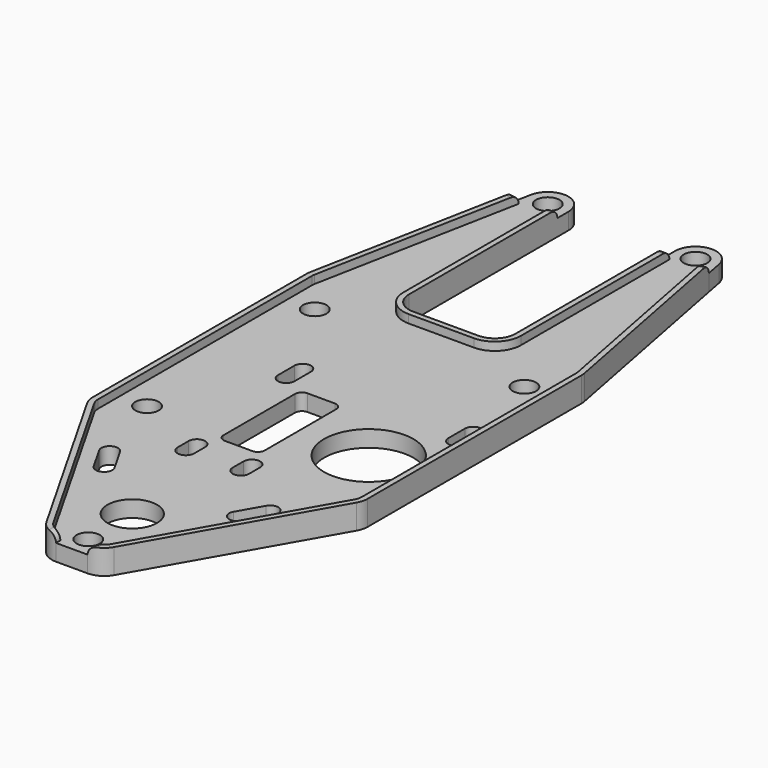
from build123d import *

# Parameters (mm, degrees)
F0_R     = 1.7
F0_R_2   = 3.6
F0_R_3   = 6.5
F1_DEPTH = 2.4
F2_DEPTH = 3.6
F3_R     = 1.19999


# Not quite as in the source:
# - a fillet or chamfer is up to 0.001 mm smaller than in the source, because OpenCascade refuses the exact size


with BuildPart() as f1:
    # F0 (on Top) → F1 (new body)
    with BuildSketch(Plane.XY):
        with BuildLine():
            Line((13.3779826676, 50), (14.1634030533, 50.1520355803))
            Line((14.1634030533, 50.1520355803), (13.6953264465, 52.5701334259))
            ThreePointArc((13.6953264465, 52.5701334259), (12.6591358938, 54.3141305363), (10.75, 55))
            ThreePointArc((10.75, 55), (8.6286796564, 54.1213203436), (7.75, 52))
            Line((7.75, 52), (7.75, 50))
            Line((7.75, 50), (8.55, 50))
            Line((8.55, 50), (8.55, 23))
            ThreePointArc((8.55, 23), (7.4370057685, 20.3129942315), (4.75, 19.2))
            Line((4.75, 19.2), (0, 19.2))
            Line((0, 19.2), (-4.75, 19.2))
            ThreePointArc((-4.75, 19.2), (-7.4370057685, 20.3129942315), (-8.55, 23))
            Line((-8.55, 23), (-8.55, 50))
            Line((-8.55, 50), (-7.75, 50))
            Line((-7.75, 50), (-7.75, 52))
            ThreePointArc((-7.75, 52), (-8.6286796564, 54.1213203436), (-10.75, 55))
            ThreePointArc((-10.75, 55), (-12.6591358938, 54.3141305363), (-13.6953264465, 52.5701334259))
            Line((-13.6953264465, 52.5701334259), (-14.1634030533, 50.1520355803))
            Line((-14.1634030533, 50.1520355803), (-13.3779826676, 50))
            Line((-13.3779826676, 50), (-19.1599060608, 20.1304096433))
            ThreePointArc((-19.1599060608, 20.1304096433), (-19.1899535764, 19.9223197335), (-19.2, 19.7123117976))
            Line((-19.2, 19.7123117976), (-19.2, 0))
            Line((-19.2, 0), (-19.2, -19.2052668078))
            ThreePointArc((-19.2, -19.2052668078), (-19.1266435215, -19.768638206), (-18.9114660616, -20.294439657))
            Line((-18.9114660616, -20.294439657), (-4.2133641117, -46.0891728492))
            ThreePointArc((-4.2133641117, -46.0891728492), (-3.4072983694, -46.9021277912), (-2.3018980501, -47.2))
            Line((-2.3018980501, -47.2), (-2.3018980501, -48))
            Line((-2.3018980501, -48), (0, -48))
            Line((0, -48), (2.3018980501, -48))
            Line((2.3018980501, -48), (2.3018980501, -47.2))
            ThreePointArc((2.3018980501, -47.2), (3.4072983694, -46.9021277912), (4.2133641117, -46.0891728492))
            Line((4.2133641117, -46.0891728492), (18.9114660616, -20.294439657))
            ThreePointArc((18.9114660616, -20.294439657), (19.1266435215, -19.768638206), (19.2, -19.2052668078))
            Line((19.2, -19.2052668078), (19.2, 0))
            Line((19.2, 0), (19.2, 19.7123117976))
            ThreePointArc((19.2, 19.7123117976), (19.1899535764, 19.9223197335), (19.1599060608, 20.1304096433))
            Line((19.1599060608, 20.1304096433), (13.3779826676, 50))
        make_face()
        with BuildLine():
            ThreePointArc((-8.6554840981, -29.4059057186), (-9.1040076685, -31.0426178518), (-10.7407198016, -30.5940942814))
            Line((-10.7407198016, -30.5940942814), (-12.721034073, -27.1187014422))
            ThreePointArc((-12.721034073, -27.1187014422), (-12.2725105026, -25.4819893091), (-10.6357983695, -25.9305128794))
            Line((-10.6357983695, -25.9305128794), (-8.6554840981, -29.4059057186))
        make_face(mode=Mode.SUBTRACT)
        with Locations((-15.25, -15.25)):
            Circle(F0_R, mode=Mode.SUBTRACT)
        with BuildLine():
            Line((-6.2, -21), (-6.2, -19))
            ThreePointArc((-6.2, -19), (-5, -17.8), (-3.8, -19))
            Line((-3.8, -19), (-3.8, -21))
            ThreePointArc((-3.8, -21), (-5, -22.2), (-6.2, -21))
        make_face(mode=Mode.SUBTRACT)
        with BuildLine():
            Line((-8.4, 0), (-8.4, 3))
            ThreePointArc((-8.4, 3), (-7.2, 4.2), (-6, 3))
            Line((-6, 3), (-6, 0))
            ThreePointArc((-6, 0), (-7.2, -1.2), (-8.4, 0))
        make_face(mode=Mode.SUBTRACT)
        with BuildLine():
            ThreePointArc((-4, -2.4), (-3.7071067812, -1.6928932188), (-3, -1.4))
            Line((-3, -1.4), (1, -1.4))
            ThreePointArc((1, -1.4), (1.7071067812, -1.6928932188), (2, -2.4))
            Line((2, -2.4), (2, -15.4))
            ThreePointArc((2, -15.4), (1.7071067812, -16.1071067812), (1, -16.4))
            Line((1, -16.4), (-3, -16.4))
            ThreePointArc((-3, -16.4), (-3.7071067812, -16.1071067812), (-4, -15.4))
            Line((-4, -15.4), (-4, -2.4))
        make_face(mode=Mode.SUBTRACT)
        with Locations((0, -45)):
            Circle(F0_R, mode=Mode.SUBTRACT)
        with Locations((0, -37)):
            Circle(F0_R_2, mode=Mode.SUBTRACT)
        with BuildLine():
            Line((12.721034073, -27.1187014422), (10.7407198016, -30.5940942814))
            ThreePointArc((10.7407198016, -30.5940942814), (9.1040076685, -31.0426178518), (8.6554840981, -29.4059057186))
            Line((8.6554840981, -29.4059057186), (10.6357983695, -25.9305128794))
            ThreePointArc((10.6357983695, -25.9305128794), (12.2725105026, -25.4819893091), (12.721034073, -27.1187014422))
        make_face(mode=Mode.SUBTRACT)
        with BuildLine():
            Line((1.8, -21), (1.8, -19))
            ThreePointArc((1.8, -19), (3, -17.8), (4.2, -19))
            Line((4.2, -19), (4.2, -21))
            ThreePointArc((4.2, -21), (3, -22.2), (1.8, -21))
        make_face(mode=Mode.SUBTRACT)
        with Locations((12, -9)):
            Circle(F0_R_3, mode=Mode.SUBTRACT)
        with BuildLine():
            Line((18.8, 3), (18.8, 0))
            ThreePointArc((18.8, 0), (17.6, -1.2), (16.4, 0))
            Line((16.4, 0), (16.4, 3))
            ThreePointArc((16.4, 3), (17.6, 4.2), (18.8, 3))
        make_face(mode=Mode.SUBTRACT)
        with Locations((-15.25, 15.25)):
            Circle(F0_R, mode=Mode.SUBTRACT)
        with Locations((-10.75, 52)):
            Circle(F0_R, mode=Mode.SUBTRACT)
        with Locations((15.25, 15.25)):
            Circle(F0_R, mode=Mode.SUBTRACT)
        with Locations((10.75, 52)):
            Circle(F0_R, mode=Mode.SUBTRACT)
    extrude(amount=F1_DEPTH)

    # F0 (on Top) → F2 (join)
    with BuildSketch(Plane.XY):
        with BuildLine():
            Line((20, -19.2052668078), (20, 0))
            Line((20, 0), (20, 19.7123117976))
            ThreePointArc((20, 19.7123117976), (19.9863003315, 19.9986862557), (19.9453264465, 20.2824452236))
            Line((19.9453264465, 20.2824452236), (14.1634030533, 50.1520355803))
            Line((14.1634030533, 50.1520355803), (13.3779826676, 50))
            Line((13.3779826676, 50), (19.1599060608, 20.1304096433))
            ThreePointArc((19.1599060608, 20.1304096433), (19.1899535764, 19.9223197335), (19.2, 19.7123117976))
            Line((19.2, 19.7123117976), (19.2, 0))
            Line((19.2, 0), (19.2, -19.2052668078))
            ThreePointArc((19.2, -19.2052668078), (19.1266435215, -19.768638206), (18.9114660616, -20.294439657))
            Line((18.9114660616, -20.294439657), (4.2133641117, -46.0891728492))
            ThreePointArc((4.2133641117, -46.0891728492), (3.4072983694, -46.9021277912), (2.3018980501, -47.2))
            Line((2.3018980501, -47.2), (2.3018980501, -48))
            ThreePointArc((2.3018980501, -48), (3.8092621219, -47.5938106244), (4.9084426795, -46.4852357035))
            Line((4.9084426795, -46.4852357035), (19.6065446294, -20.6905025113))
            ThreePointArc((19.6065446294, -20.6905025113), (19.8999684385, -19.9735005326), (20, -19.2052668078))
        make_face()
        with BuildLine():
            Line((8.55, 50), (7.75, 50))
            Line((7.75, 50), (7.75, 23))
            ThreePointArc((7.75, 23), (6.8713203436, 20.8786796564), (4.75, 20))
            Line((4.75, 20), (0, 20))
            Line((0, 20), (-4.75, 20))
            ThreePointArc((-4.75, 20), (-6.8713203436, 20.8786796564), (-7.75, 23))
            Line((-7.75, 23), (-7.75, 50))
            Line((-7.75, 50), (-8.55, 50))
            Line((-8.55, 50), (-8.55, 23))
            ThreePointArc((-8.55, 23), (-7.4370057685, 20.3129942315), (-4.75, 19.2))
            Line((-4.75, 19.2), (0, 19.2))
            Line((0, 19.2), (4.75, 19.2))
            ThreePointArc((4.75, 19.2), (7.4370057685, 20.3129942315), (8.55, 23))
            Line((8.55, 23), (8.55, 50))
        make_face()
        with BuildLine():
            ThreePointArc((-4.9084426795, -46.4852357035), (-3.8092621219, -47.5938106244), (-2.3018980501, -48))
            Line((-2.3018980501, -48), (-2.3018980501, -47.2))
            ThreePointArc((-2.3018980501, -47.2), (-3.4072983694, -46.9021277912), (-4.2133641117, -46.0891728492))
            Line((-4.2133641117, -46.0891728492), (-18.9114660616, -20.294439657))
            ThreePointArc((-18.9114660616, -20.294439657), (-19.1266435215, -19.768638206), (-19.2, -19.2052668078))
            Line((-19.2, -19.2052668078), (-19.2, 0))
            Line((-19.2, 0), (-19.2, 19.7123117976))
            ThreePointArc((-19.2, 19.7123117976), (-19.1899535764, 19.9223197335), (-19.1599060608, 20.1304096433))
            Line((-19.1599060608, 20.1304096433), (-13.3779826676, 50))
            Line((-13.3779826676, 50), (-14.1634030533, 50.1520355803))
            Line((-14.1634030533, 50.1520355803), (-19.9453264465, 20.2824452236))
            ThreePointArc((-19.9453264465, 20.2824452236), (-19.9863003315, 19.9986862557), (-20, 19.7123117976))
            Line((-20, 19.7123117976), (-20, 0))
            Line((-20, 0), (-20, -19.2052668078))
            ThreePointArc((-20, -19.2052668078), (-19.8999684385, -19.9735005326), (-19.6065446294, -20.6905025113))
            Line((-19.6065446294, -20.6905025113), (-4.9084426795, -46.4852357035))
        make_face()
    extrude(amount=F2_DEPTH)

    # F3 (radius 1.2 in the source; OpenCascade refuses exactly that, so slightly less here)
    f3_edges = [f1.edges().sort_by_distance(p)[0] for p in [
        (-13.770693, 50.076018, 3.6),
        (-8.15, 50, 3.6),
        (8.15, 50, 3.6),
        (13.770693, 50.076018, 3.6),
        (-2.301898, -47.6, 3.6),
        (2.301898, -47.6, 3.6),
    ]]
    fillet(f3_edges, radius=F3_R)


solid = f1.part
